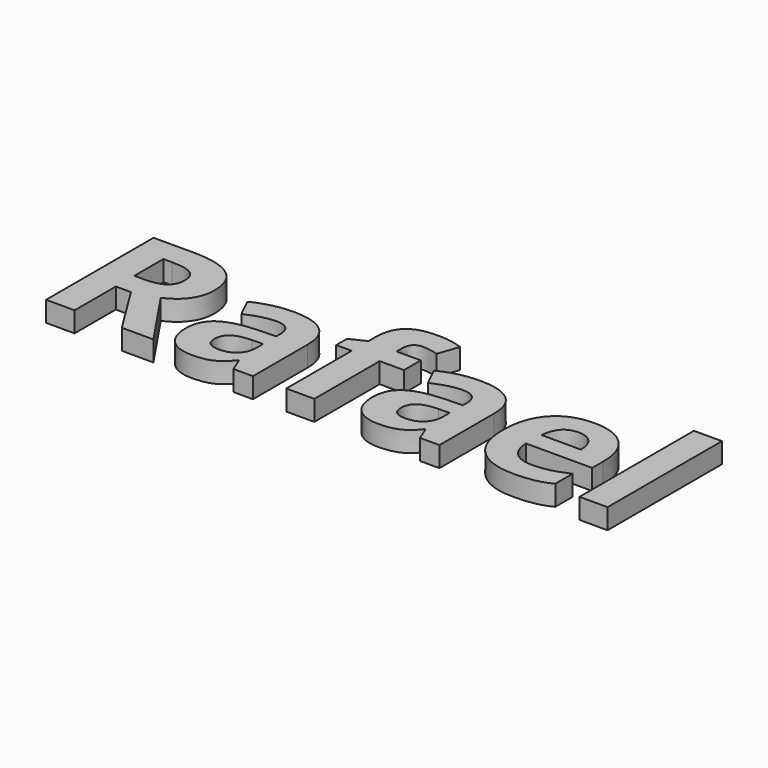
from build123d import *

# Parameters (mm, degrees)
F0_TEXT_SIZE = 27.7777777778
F1_DEPTH     = 3


# Not quite as in the source:
# - Text() gives the source's letters only with a copy of the font that has no kerning and outlines rounded to 1/6400 em; it was checked with that copy


with BuildPart() as f1:
    # F0 (on Top) → F1 (new body)
    with BuildSketch(Plane.XY):
        with Locations((-32.1603268091, -9.8976548226)):
            Text('Rafael', F0_TEXT_SIZE, font='Open Sans', font_style=FontStyle.BOLD, text_align=(TextAlign.LEFT, TextAlign.BOTTOM))
    extrude(amount=F1_DEPTH)


solid = f1.part
